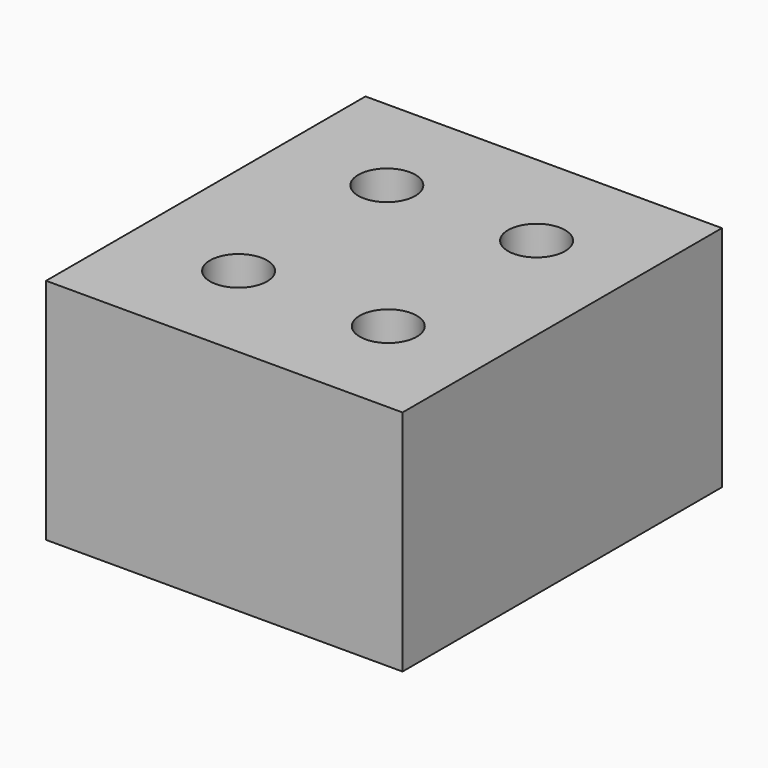
from build123d import *

# Parameters (mm, degrees)
F0_W     = 28
F0_H     = 28
F1_DEPTH = 16
F3_D     = 4
F4_DEPTH = 3


with BuildPart() as f1:
    # F0 (on Top) → F1 (new body)
    with BuildSketch(Plane.XY):
        Rectangle(F0_W, F0_H)
    extrude(amount=F1_DEPTH)

    # F3 (through all)
    with Locations(Plane.XY.offset(16)):
        with Locations((4, -6.5), (-6.5, -6.5), (-6.5, 6.5), (4, 6.5)):
            Hole(F3_D / 2)

    # F4 (cut): a face of the model
    f4_faces = [f1.faces().sort_by_distance(p)[0] for p in [
        (14, 0, 8),
    ]]
    extrude(f4_faces, amount=-F4_DEPTH, mode=Mode.SUBTRACT)


solid = f1.part
